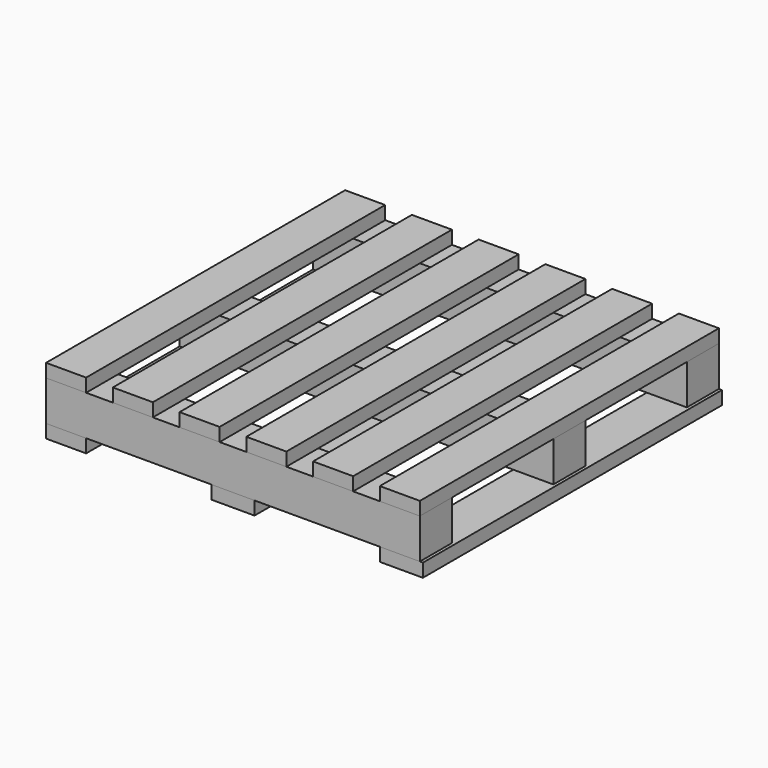
from build123d import *

# Parameters (mm, degrees)
F1_W          = 9.525
F1_H          = 88.9
F2_DEPTH      = 3.175
F3_W          = 9.525
F3_H          = 9.525
F4_DEPTH      = 44.45
F4_DEPTH_BACK = 44.45
F5_W          = 10.2447643876
F5_H          = 88.9
F6_DEPTH      = 3.175
F5_W_2        = 9.5249999999


# Not quite as in the source:
# - a variable given as a bare number and used for a length is read in inches; the dataset says mm whatever the document's units were


with BuildPart() as f2:
    # F1 (on Top) → F2 (new body)
    with BuildSketch(Plane.XY):
        with Locations((-39.6875, 0)):
            Rectangle(F1_W, F1_H)
    extrude(amount=F2_DEPTH)


with BuildPart() as f2b:
    # F1 (on Top) → F2, piece 2 (new body)
    with BuildSketch(Plane.XY):
        with Locations((-23.8125, 0)):
            Rectangle(F1_W, F1_H)
    extrude(amount=F2_DEPTH)


with BuildPart() as f2c:
    # F1 (on Top) → F2, piece 3 (new body)
    with BuildSketch(Plane.XY):
        with Locations((-7.9375, 0)):
            Rectangle(F1_W, F1_H)
    extrude(amount=F2_DEPTH)


with BuildPart() as f2d:
    # F1 (on Top) → F2, piece 4 (new body)
    with BuildSketch(Plane.XY):
        with Locations((7.9375, 0)):
            Rectangle(F1_W, F1_H)
    extrude(amount=F2_DEPTH)


with BuildPart() as f2e:
    # F1 (on Top) → F2, piece 5 (new body)
    with BuildSketch(Plane.XY):
        with Locations((23.8125, 0)):
            Rectangle(F1_W, F1_H)
    extrude(amount=F2_DEPTH)


with BuildPart() as f2f:
    # F1 (on Top) → F2, piece 6 (new body)
    with BuildSketch(Plane.XY):
        with Locations((39.6875, 0)):
            Rectangle(F1_W, F1_H)
    extrude(amount=F2_DEPTH)


with BuildPart() as f4:
    # F3 (on Right) → F4 (new body, two sides)
    with BuildSketch(Plane.YZ) as f4_sk:
        with Locations((-39.6875, -4.7625)):
            Rectangle(F3_W, F3_H)
    extrude(amount=F4_DEPTH)
    extrude(f4_sk.sketch, amount=-F4_DEPTH_BACK)


with BuildPart() as f4b:
    # F3 (on Right) → F4, piece 2 (new body, two sides)
    with BuildSketch(Plane.YZ) as f4_2_sk:
        with Locations((39.6875, -4.7625)):
            Rectangle(F3_W, F3_H)
    extrude(amount=F4_DEPTH)
    extrude(f4_2_sk.sketch, amount=-F4_DEPTH_BACK)


with BuildPart() as f4c:
    # F3 (on Right) → F4, piece 3 (new body, two sides)
    with BuildSketch(Plane.YZ) as f4_3_sk:
        with Locations((0, -4.7625)):
            Rectangle(F3_W, F3_H)
    extrude(amount=F4_DEPTH)
    extrude(f4_3_sk.sketch, amount=-F4_DEPTH_BACK)


with BuildPart() as f6:
    # F5 (on face) → F6 (new body)
    with BuildSketch(Plane(origin=(0, 0, -9.525), x_dir=(1, 0, 0), z_dir=(0, 0, -1))):
        with Locations((40.0473821938, 0)):
            Rectangle(F5_W, F5_H)
    extrude(amount=F6_DEPTH)


with BuildPart() as f6b:
    # F5 (on face) → F6, piece 2 (new body)
    with BuildSketch(Plane(origin=(0, 0, -9.525), x_dir=(1, 0, 0), z_dir=(0, 0, -1))):
        with Locations((-39.6874999999, 0)):
            Rectangle(F5_W_2, F5_H)
    extrude(amount=F6_DEPTH)


with BuildPart() as f6c:
    # F5 (on face) → F6, piece 3 (new body)
    with BuildSketch(Plane(origin=(0, 0, -9.525), x_dir=(1, 0, 0), z_dir=(0, 0, -1))):
        Rectangle(F5_W, F5_H)
    extrude(amount=F6_DEPTH)


solid = Compound([f2.part, f2b.part, f2c.part, f2d.part, f2e.part, f2f.part, f4.part, f4b.part, f4c.part, f6.part, f6b.part, f6c.part])
